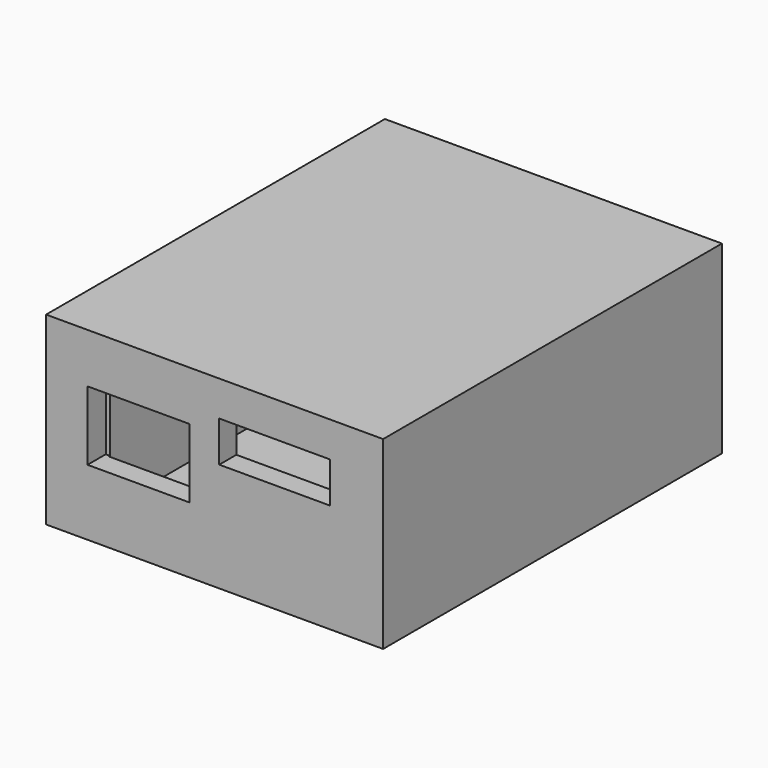
from build123d import *

# Parameters (mm, degrees)
F0_W         = 42.1587601304
F0_H         = 52.9734008014
F0_W_2       = 34.925
F0_H_2       = 47.625
F1_DEPTH     = 18.034
F2_DEPTH     = 2.54
F3_W         = 34.925
F3_H         = 18.034
F2_FACE_W    = 42.1587601304
F2_FACE_H    = 20.574
F4_DEPTH     = 10.32974
F5_W         = 42.1587601304
F5_H         = 52.9734008014
F6_DEPTH     = 2.54
F7_W         = 13.8736660592
F7_H         = 5.0836820155
F8_DEPTH     = 25.4
F9_W         = 6.2576979399
F9_H         = 1.2498646975
F10_DEPTH    = 0.635
F11_T1_DEPTH = 10.2510766125
F12_DEPTH    = 2.0923395641
F13_W        = 12.7831122372
F13_H        = 8.6434278637
F14_DEPTH    = 2.8529665433


# Not quite as in the source:
# - a fillet or chamfer that OpenCascade refuses, or shapes differently, is made with other operations: its cross-section is extruded or revolved along the edge and cut away or added


with BuildPart() as f1:
    # F0 (on Top) → F1 (new body)
    with BuildSketch(Plane.XY):
        Rectangle(F0_W, F0_H)
        Rectangle(F0_W_2, F0_H_2, mode=Mode.SUBTRACT)
    extrude(amount=F1_DEPTH)

    # F0 (on Top) → F2 (join)
    with BuildSketch(Plane.XY):
        Rectangle(F0_W, F0_H)
        Rectangle(F0_W_2, F0_H_2, mode=Mode.SUBTRACT)
        Rectangle(F0_W_2, F0_H_2)
    extrude(amount=-F2_DEPTH)

    # F3 (on face) + F2_face (on face) → F4 (cut)
    with BuildSketch(Plane.XZ.offset(-23.8125)):
        with Locations((0, 9.017)):
            Rectangle(F3_W, F3_H)
    with BuildSketch(Plane(origin=(0, 26.4867004007, 7.747), x_dir=(-1, 0, 0), z_dir=(0, 1, 0))):
        Rectangle(F2_FACE_W, F2_FACE_H)
    extrude(amount=-F4_DEPTH, dir=(0, -1, 0), mode=Mode.SUBTRACT)

    # F5 (on face) → F6 (join)
    with BuildSketch(Plane.XY.offset(18.034)):
        Rectangle(F5_W, F5_H)
    extrude(amount=F6_DEPTH)

    # F7 (on face) → F8 (cut)
    with BuildSketch(Plane.XZ.offset(26.4867004007)):
        with Locations((7.517300779, 13.6317610741)):
            Rectangle(F7_W, F7_H)
    extrude(amount=-F8_DEPTH, mode=Mode.SUBTRACT)

    # F9 (on face) → F10 (join)
    with BuildSketch(Plane.XY):
        with Locations((0, 25.5755782127)):
            Rectangle(F9_W, F9_H)
    extrude(amount=F10_DEPTH)

    # F11: fillet of radius 0.8197700228 on 2 edges, made by hand

    # F11_s2 → F11_t1 (cut)
    with BuildSketch(Plane.YZ.offset(-5.1255383063)):
        with BuildLine():
            ThreePointArc((26.2005105615, 0), (25.9120083094, 0.4569042778), (25.4018348269, 0.635))
            Line((25.4018348269, 0.635), (26.2005105615, 0.635))
            Line((26.2005105615, 0.635), (26.2005105615, 0))
        make_face()
        with BuildLine():
            ThreePointArc((24.950645864, 0), (25.2391481161, 0.4569042778), (25.7493215985, 0.635))
            Line((25.7493215985, 0.635), (24.950645864, 0.635))
            Line((24.950645864, 0.635), (24.950645864, 0))
        make_face()
    extrude(amount=F11_T1_DEPTH, mode=Mode.SUBTRACT)

    # F12 (add): a face of the model
    f12_faces = [f1.faces().sort_by_distance(p)[0] for p in [
        (-17.4625, 1.3371002004, 9.017),
    ]]
    extrude(f12_faces, amount=F12_DEPTH)

    # F13 (on face) → F14 (cut)
    with BuildSketch(Plane.XZ.offset(26.4867004007)):
        with Locations((-9.5031157834, 10.0388908759)):
            Rectangle(F13_W, F13_H)
    extrude(amount=-F14_DEPTH, mode=Mode.SUBTRACT)


solid = f1.part
